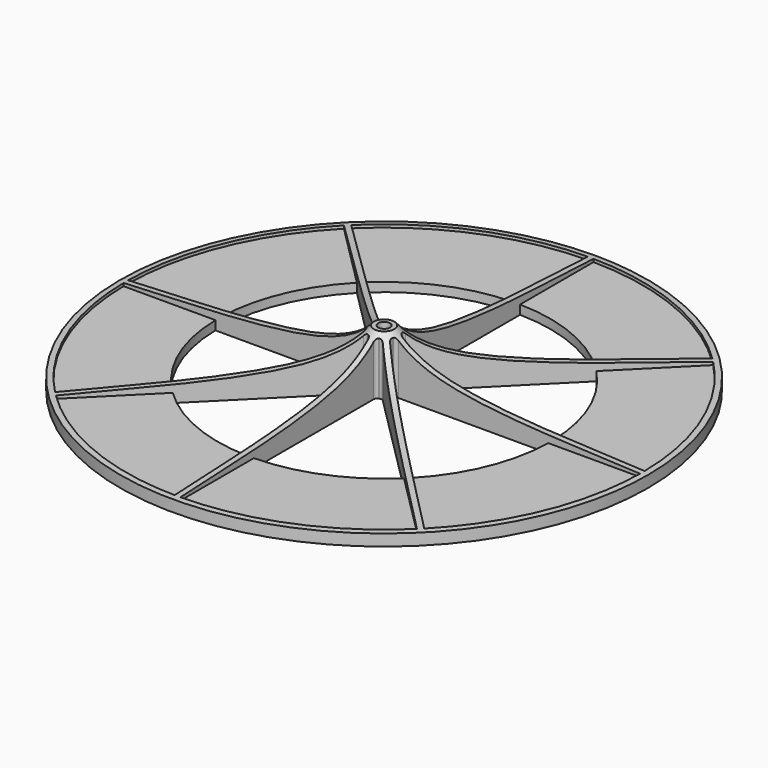
from build123d import *

# Parameters (mm, degrees)
F0_R     = 58.42
F0_R_2   = 1.3081
F1_DEPTH = 12.7
F2_R     = 58.42
F2_R_2   = 36.83
F3_DEPTH = 2


# Not quite as in the source:
# - a feature names something its author has since deleted; it is built from what else it names


with BuildPart() as f1:
    # F0 (on Top) → F1 (new body)
    with BuildSketch(Plane.XY):
        Circle(F0_R)
        with BuildLine():
            ThreePointArc((-0.635, -57.1464721133), (-21.8703581597, -52.799715283), (-39.9596451462, -40.8576707583))
            Line((-39.9596451462, -40.8576707583), (-27.3861598627, -28.2841854748))
            Line((-27.3861598627, -28.2841854748), (-2.1537126885, -3.0517383006))
            ThreePointArc((-2.1537126885, -3.0517383006), (-1.7523453807, -2.8410524798), (-1.3023365494, -2.8956077967))
            ThreePointArc((-1.3023365494, -2.8956077967), (-1.2150198978, -2.9333175157), (-1.1266129032, -2.9683949141))
            ThreePointArc((-1.1266129032, -2.9683949141), (-0.7698321725, -3.2480227758), (-0.635, -3.6808096935))
            Line((-0.635, -3.6808096935), (-0.635, -38.0947079658))
            Line((-0.635, -38.0947079658), (-0.635, -57.1464721133))
        make_face(mode=Mode.SUBTRACT)
        with BuildLine():
            ThreePointArc((-40.8576707583, -39.9596451462), (-52.799715283, -21.8703581597), (-57.1464721133, -0.635))
            Line((-57.1464721133, -0.635), (-39.3648786992, -0.635))
            Line((-39.3648786992, -0.635), (-3.6808096935, -0.635))
            ThreePointArc((-3.6808096935, -0.635), (-3.2480227758, -0.7698321725), (-2.9683949141, -1.1266129032))
            ThreePointArc((-2.9683949141, -1.1266129032), (-2.9333175157, -1.2150198978), (-2.8956077967, -1.3023365494))
            ThreePointArc((-2.8956077967, -1.3023365494), (-2.8410524798, -1.7523453807), (-3.0517383006, -2.1537126885))
            Line((-3.0517383006, -2.1537126885), (-27.386039136, -26.4880135239))
            Line((-27.386039136, -26.4880135239), (-40.8576707583, -39.9596451462))
        make_face(mode=Mode.SUBTRACT)
        Circle(F0_R_2, mode=Mode.SUBTRACT)
        with BuildLine():
            ThreePointArc((39.9596451462, -40.8576707583), (21.8703581597, -52.799715283), (0.635, -57.1464721133))
            Line((0.635, -57.1464721133), (0.635, -39.3648786992))
            Line((0.635, -39.3648786992), (0.635, -3.6808096935))
            ThreePointArc((0.635, -3.6808096935), (0.7698321725, -3.2480227758), (1.1266129032, -2.9683949141))
            ThreePointArc((1.1266129032, -2.9683949141), (1.2150198978, -2.9333175157), (1.3023365494, -2.8956077967))
            ThreePointArc((1.3023365494, -2.8956077967), (1.7523453807, -2.8410524798), (2.1537126885, -3.0517383006))
            Line((2.1537126885, -3.0517383006), (27.3861598627, -28.2841854748))
            Line((27.3861598627, -28.2841854748), (39.9596451462, -40.8576707583))
        make_face(mode=Mode.SUBTRACT)
        with BuildLine():
            ThreePointArc((57.1464721133, -0.635), (52.799715283, -21.8703581597), (40.8576707583, -39.9596451462))
            Line((40.8576707583, -39.9596451462), (27.386039136, -26.4880135239))
            Line((27.386039136, -26.4880135239), (3.0517383006, -2.1537126885))
            ThreePointArc((3.0517383006, -2.1537126885), (2.8410524798, -1.7523453807), (2.8956077967, -1.3023365494))
            ThreePointArc((2.8956077967, -1.3023365494), (2.9333175157, -1.2150198978), (2.9683949141, -1.1266129032))
            ThreePointArc((2.9683949141, -1.1266129032), (3.2480227758, -0.7698321725), (3.6808096935, -0.635))
            Line((3.6808096935, -0.635), (38.0947079658, -0.635))
            Line((38.0947079658, -0.635), (57.1464721133, -0.635))
        make_face(mode=Mode.SUBTRACT)
        with BuildLine():
            ThreePointArc((-3.0517383006, 2.1537126885), (-2.8410524798, 1.7523453807), (-2.8956077967, 1.3023365494))
            ThreePointArc((-2.8956077967, 1.3023365494), (-2.9333175157, 1.2150198978), (-2.9683949141, 1.1266129032))
            ThreePointArc((-2.9683949141, 1.1266129032), (-3.2480227758, 0.7698321725), (-3.6808096935, 0.635))
            Line((-3.6808096935, 0.635), (-38.0947079658, 0.635))
            Line((-38.0947079658, 0.635), (-57.1464721133, 0.635))
            ThreePointArc((-57.1464721133, 0.635), (-52.799715283, 21.8703581597), (-40.8576707583, 39.9596451462))
            Line((-40.8576707583, 39.9596451462), (-27.386039136, 26.4880135239))
            Line((-27.386039136, 26.4880135239), (-3.0517383006, 2.1537126885))
        make_face(mode=Mode.SUBTRACT)
        with BuildLine():
            ThreePointArc((-39.9596451462, 40.8576707583), (-21.8703581597, 52.799715283), (-0.635, 57.1464721133))
            Line((-0.635, 57.1464721133), (-0.635, 39.3648786992))
            Line((-0.635, 39.3648786992), (-0.635, 3.6808096935))
            ThreePointArc((-0.635, 3.6808096935), (-0.7698321725, 3.2480227758), (-1.1266129032, 2.9683949141))
            ThreePointArc((-1.1266129032, 2.9683949141), (-1.2150198978, 2.9333175157), (-1.3023365494, 2.8956077967))
            ThreePointArc((-1.3023365494, 2.8956077967), (-1.7523453807, 2.8410524798), (-2.1537126885, 3.0517383006))
            Line((-2.1537126885, 3.0517383006), (-26.4880135239, 27.386039136))
            Line((-26.4880135239, 27.386039136), (-39.9596451462, 40.8576707583))
        make_face(mode=Mode.SUBTRACT)
        with BuildLine():
            ThreePointArc((40.8576707583, 39.9596451462), (52.799715283, 21.8703581597), (57.1464721133, 0.635))
            Line((57.1464721133, 0.635), (39.3648786992, 0.635))
            Line((39.3648786992, 0.635), (3.6808096935, 0.635))
            ThreePointArc((3.6808096935, 0.635), (3.2480227758, 0.7698321725), (2.9683949141, 1.1266129032))
            ThreePointArc((2.9683949141, 1.1266129032), (2.9333175157, 1.2150198978), (2.8956077967, 1.3023365494))
            ThreePointArc((2.8956077967, 1.3023365494), (2.8410524798, 1.7523453807), (3.0517383006, 2.1537126885))
            Line((3.0517383006, 2.1537126885), (28.2841854748, 27.3861598627))
            Line((28.2841854748, 27.3861598627), (40.8576707583, 39.9596451462))
        make_face(mode=Mode.SUBTRACT)
        with BuildLine():
            Line((0.635, 38.0947079658), (0.635, 57.1464721133))
            ThreePointArc((0.635, 57.1464721133), (21.8703581597, 52.799715283), (39.9596451462, 40.8576707583))
            Line((39.9596451462, 40.8576707583), (26.4880135239, 27.386039136))
            Line((26.4880135239, 27.386039136), (2.1537126885, 3.0517383006))
            ThreePointArc((2.1537126885, 3.0517383006), (1.7523453807, 2.8410524798), (1.3023365494, 2.8956077967))
            ThreePointArc((1.3023365494, 2.8956077967), (1.2150198978, 2.9333175157), (1.1266129032, 2.9683949141))
            ThreePointArc((1.1266129032, 2.9683949141), (0.7698321725, 3.2480227758), (0.635, 3.6808096935))
            Line((0.635, 3.6808096935), (0.635, 38.0947079658))
        make_face(mode=Mode.SUBTRACT)
    extrude(amount=F1_DEPTH)

    # F2 (on Top) → F3 (join)
    with BuildSketch(Plane.XY):
        Circle(F2_R)
        Circle(F2_R_2, mode=Mode.SUBTRACT)
    extrude(amount=F3_DEPTH)

    # F4 (on Right) → F5 (revolve, cut)
    with BuildSketch(Plane.YZ):
        with BuildLine():
            Line((63.2786378264, 24.0727756172), (0, 24.0727756172))
            Line((0, 24.0727756172), (0, 16.6299855337))
            add(Edge.make_bspline(
                [(0, 16.6299855337), (1.6776970372, 12.1904821945), (11.5130469036, 2.3314553589), (63.1935885893, 3.5681672558), (63.0198984491, 1.3907300471), (63.2786378264, 0)],
                knots=[0, 0, 0, 0, 0.3291428863, 0.8747545175, 1, 1, 1, 1], degree=3))
            Line((63.2786378264, 0), (63.2786378264, 24.0727756172))
        make_face()
    revolve(axis=Axis((0, 0, 0), (0, 0, -1)), mode=Mode.SUBTRACT)


solid = f1.part
